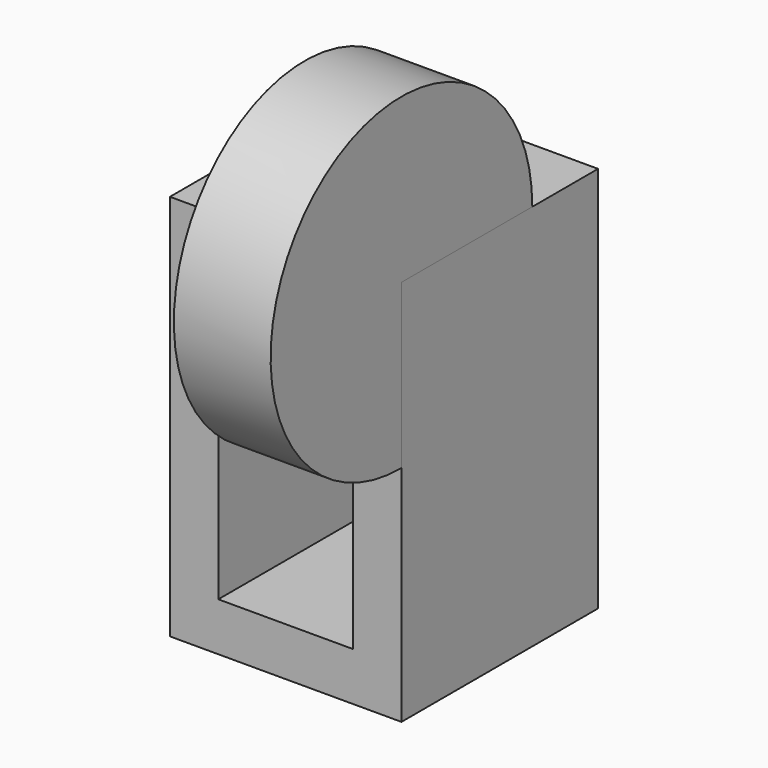
from build123d import *

# Parameters (mm, degrees)
F0_W     = 60.7822282831
F0_H     = 64.516
F1_DEPTH = 101.6
F2_T     = -12.7
F4_DEPTH = 25.4


with BuildPart() as f1:
    # F0 (on Top) → F1 (new body)
    with BuildSketch(Plane.XY):
        Rectangle(F0_W, F0_H)
    extrude(amount=F1_DEPTH)

    # F2
    f2_openings = [f1.faces().sort_by_distance(p)[0] for p in [
        (0, -32.258, 50.8),
    ]]
    offset(amount=F2_T, openings=f2_openings)


with BuildPart() as f4:
    # F3 (on face) → F4 (new body)
    with BuildSketch(Plane.YZ.offset(30.3911141416)):
        with BuildLine():
            Line((-32.258, 101.6), (10.6755790953, 101.6))
            ThreePointArc((10.6755790953, 101.6), (-62.6166249189, 131.9586249189), (-32.258, 58.6664209047))
            Line((-32.258, 58.6664209047), (-32.258, 101.6))
        make_face()
    extrude(amount=-F4_DEPTH)


solid = Compound([f1.part, f4.part])
